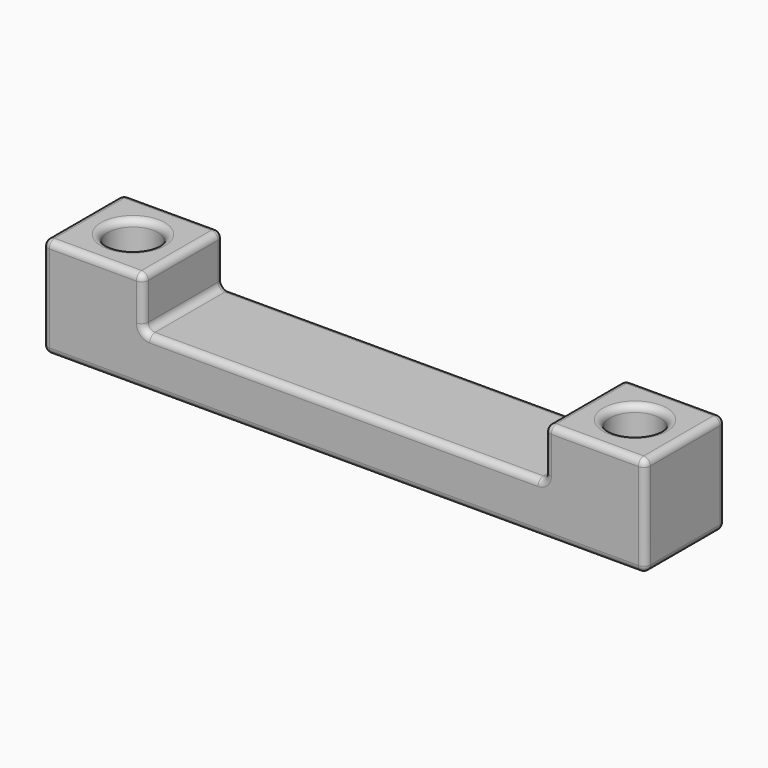
from build123d import *

# Parameters (mm, degrees)
F1_DEPTH      = 19.05
F2_R          = 4.7625
F3_DEPTH      = 19.051
F4_R          = 7.9375
F4_R_2        = 4.7625
F5_DEPTH      = 6.35
F6_T1_DEPTH   = 19.05
F6_T3_DEPTH   = 16.51
F6_T5_DEPTH   = 111.76
F6_T7_DEPTH   = 20.955
F6_T9_DEPTH   = 20.955
F6_T11_DEPTH  = 16.51
F6_T13_DEPTH  = 25.4
F6_S17_W      = 1.27
F6_S17_H      = 1.27
F6_T18_DEPTH  = 1.27
F6_S23_W      = 1.27
F6_S23_H      = 1.27
F6_T24_DEPTH  = 1.27
F6_S29_W      = 1.27
F6_S29_H      = 1.27
F6_T30_DEPTH  = 1.27
F6_S35_W      = 1.27
F6_S35_H      = 1.27
F6_T36_DEPTH  = 1.27
F6_S41_W      = 1.27
F6_S41_H      = 1.27
F6_T42_DEPTH  = 1.27
F6_S47_W      = 1.27
F6_S47_H      = 1.27
F6_T48_DEPTH  = 1.27
F6_S53_W      = 1.27
F6_S53_H      = 1.27
F6_T54_DEPTH  = 1.27
F6_S59_W      = 1.27
F6_S59_H      = 1.27
F6_T60_DEPTH  = 1.27
F6_T71_DEPTH  = 6.985
F6_T73_DEPTH  = 73.66
F6_S77_W      = 1.27
F6_S77_H      = 1.27
F6_T78_DEPTH  = 1.27
F6_S83_W      = 1.27
F6_S83_H      = 1.27
F6_T84_DEPTH  = 1.27
F6_S89_W      = 1.27
F6_S89_H      = 1.27
F6_T90_DEPTH  = 1.27
F6_S95_W      = 1.27
F6_S95_H      = 1.27
F6_T96_DEPTH  = 1.27
F6_T100_ANGLE = 90
F6_T102_ANGLE = 90
F6_T104_ANGLE = 90
F6_T106_ANGLE = 90


# Not quite as in the source:
# - a fillet or chamfer that OpenCascade refuses, or shapes differently, is made with other operations: its cross-section is extruded or revolved along the edge and cut away or added


with BuildPart() as f1:
    # F0 (on Front) → F1 (new body)
    with BuildSketch(Plane.XZ):
        Polygon((-57.15, 19.05), (-57.15, 0), (0, 0), (57.15, 0), (57.15, 19.05), (38.1, 19.05), (38.1, 9.525), (-38.1, 9.525), (-38.1, 19.05), align=None)
    extrude(amount=F1_DEPTH)

    # F2 (on face) → F3 (cut, through all)
    with BuildSketch(Plane.XY.offset(19.05)):
        with Locations((-47.625, -9.525)):
            Circle(F2_R)
        with Locations((47.625, -9.525)):
            Circle(F2_R)
    extrude(amount=-F3_DEPTH, mode=Mode.SUBTRACT)

    # F4 (on face) → F5 (cut)
    with BuildSketch(Plane(origin=(0, 0, 0), x_dir=(1, 0, 0), z_dir=(0, 0, -1))):
        with Locations((-47.625, 9.525)):
            Circle(F4_R)
        with Locations((-47.625, 9.525)):
            Circle(F4_R_2, mode=Mode.SUBTRACT)
        with Locations((47.625, 9.525)):
            Circle(F4_R)
        with Locations((47.625, 9.525)):
            Circle(F4_R_2, mode=Mode.SUBTRACT)
    extrude(amount=-F5_DEPTH, mode=Mode.SUBTRACT)

    # F6: fillet of radius 1.27 on 28 edges, made by hand

    # F6_s2 → F6_t1 (join)
    with BuildSketch(Plane.XZ):
        with BuildLine():
            ThreePointArc((38.1, 10.795), (37.7280256121, 9.8969743879), (36.83, 9.525))
            Line((36.83, 9.525), (38.1, 9.525))
            Line((38.1, 9.525), (38.1, 10.795))
        make_face()
        with BuildLine():
            ThreePointArc((-38.1, 10.795), (-37.7280256121, 9.8969743879), (-36.83, 9.525))
            Line((-36.83, 9.525), (-38.1, 9.525))
            Line((-38.1, 9.525), (-38.1, 10.795))
        make_face()
    extrude(amount=F6_T1_DEPTH)

    # F6_s4 → F6_t3 (cut)
    with BuildSketch(Plane.XY.offset(1.27)):
        with BuildLine():
            ThreePointArc((-57.15, -17.78), (-56.7780256121, -18.6780256121), (-55.88, -19.05))
            Line((-55.88, -19.05), (-57.15, -19.05))
            Line((-57.15, -19.05), (-57.15, -17.78))
        make_face()
        with BuildLine():
            ThreePointArc((55.88, -19.05), (56.7780256121, -18.6780256121), (57.15, -17.78))
            Line((57.15, -17.78), (57.15, -19.05))
            Line((57.15, -19.05), (55.88, -19.05))
        make_face()
        with BuildLine():
            ThreePointArc((-57.15, -1.27), (-56.7780256121, -0.3719743879), (-55.88, 0))
            Line((-55.88, 0), (-57.15, 0))
            Line((-57.15, 0), (-57.15, -1.27))
        make_face()
        with BuildLine():
            ThreePointArc((55.88, 0), (56.7780256121, -0.3719743879), (57.15, -1.27))
            Line((57.15, -1.27), (57.15, 0))
            Line((57.15, 0), (55.88, 0))
        make_face()
    extrude(amount=F6_T3_DEPTH, mode=Mode.SUBTRACT)

    # F6_s6 → F6_t5 (cut)
    with BuildSketch(Plane.YZ.offset(-55.88)):
        with BuildLine():
            ThreePointArc((-17.78, 0), (-18.6780256121, 0.3719743879), (-19.05, 1.27))
            Line((-19.05, 1.27), (-19.05, 0))
            Line((-19.05, 0), (-17.78, 0))
        make_face()
        with BuildLine():
            ThreePointArc((-1.27, 0), (-0.3719743879, 0.3719743879), (0, 1.27))
            Line((0, 1.27), (0, 0))
            Line((0, 0), (-1.27, 0))
        make_face()
    extrude(amount=F6_T5_DEPTH, mode=Mode.SUBTRACT)

    # F6_s8 → F6_t7 (cut)
    with BuildSketch(Plane.YZ.offset(34.925)):
        with BuildLine():
            ThreePointArc((-19.05, 17.78), (-18.6780256121, 18.6780256121), (-17.78, 19.05))
            Line((-17.78, 19.05), (-19.05, 19.05))
            Line((-19.05, 19.05), (-19.05, 17.78))
        make_face()
        with BuildLine():
            ThreePointArc((0, 17.78), (-0.3719743879, 18.6780256121), (-1.27, 19.05))
            Line((-1.27, 19.05), (0, 19.05))
            Line((0, 19.05), (0, 17.78))
        make_face()
    extrude(amount=F6_T7_DEPTH, mode=Mode.SUBTRACT)

    # F6_s10 → F6_t9 (cut)
    with BuildSketch(Plane.YZ.offset(-55.88)):
        with BuildLine():
            ThreePointArc((-17.78, 19.05), (-18.6780256121, 18.6780256121), (-19.05, 17.78))
            Line((-19.05, 17.78), (-19.05, 19.05))
            Line((-19.05, 19.05), (-17.78, 19.05))
        make_face()
        with BuildLine():
            ThreePointArc((-1.27, 19.05), (-0.3719743879, 18.6780256121), (0, 17.78))
            Line((0, 17.78), (0, 19.05))
            Line((0, 19.05), (-1.27, 19.05))
        make_face()
    extrude(amount=F6_T9_DEPTH, mode=Mode.SUBTRACT)

    # F6_s12 → F6_t11 (cut)
    with BuildSketch(Plane.XZ.offset(1.27)):
        with BuildLine():
            ThreePointArc((57.15, 17.78), (56.7780256121, 18.6780256121), (55.88, 19.05))
            Line((55.88, 19.05), (57.15, 19.05))
            Line((57.15, 19.05), (57.15, 17.78))
        make_face()
        with BuildLine():
            ThreePointArc((-57.15, 17.78), (-56.7780256121, 18.6780256121), (-55.88, 19.05))
            Line((-55.88, 19.05), (-57.15, 19.05))
            Line((-57.15, 19.05), (-57.15, 17.78))
        make_face()
        with BuildLine():
            ThreePointArc((-57.15, 1.27), (-56.7780256121, 0.3719743879), (-55.88, 0))
            Line((-55.88, 0), (-57.15, 0))
            Line((-57.15, 0), (-57.15, 1.27))
        make_face()
        with BuildLine():
            ThreePointArc((55.88, 0), (56.7780256121, 0.3719743879), (57.15, 1.27))
            Line((57.15, 1.27), (57.15, 0))
            Line((57.15, 0), (55.88, 0))
        make_face()
    extrude(amount=F6_T11_DEPTH, mode=Mode.SUBTRACT)

    # F6_s14 → F6_t13 (cut)
    with BuildSketch(Plane.XZ.offset(-3.175)):
        with BuildLine():
            ThreePointArc((39.37, 19.05), (38.4719743879, 18.6780256121), (38.1, 17.78))
            Line((38.1, 17.78), (38.1, 19.05))
            Line((38.1, 19.05), (39.37, 19.05))
        make_face()
        with BuildLine():
            ThreePointArc((-39.37, 19.05), (-38.4719743879, 18.6780256121), (-38.1, 17.78))
            Line((-38.1, 17.78), (-38.1, 19.05))
            Line((-38.1, 19.05), (-39.37, 19.05))
        make_face()
    extrude(amount=F6_T13_DEPTH, mode=Mode.SUBTRACT)


with BuildPart() as f6_tool16:
    # F6_s17 → F6_t18 (new body)
    with BuildSketch(Plane.YZ.offset(-55.88)):
        with Locations((-18.415, 18.415)):
            Rectangle(F6_S17_W, F6_S17_H)
    extrude(amount=-F6_T18_DEPTH)

    # F6_s19 → F6_t20 (revolve, cut)
    with BuildSketch(Plane(origin=(-55.88, -17.78, 17.78), x_dir=(0, 0.7071067812, -0.7071067812), z_dir=(0, 0.7071067812, 0.7071067812))):
        with BuildLine():
            ThreePointArc((0, -1.27), (1.27, 0), (0, 1.27))
            Line((0, 1.27), (0, -1.27))
        make_face()
    revolve(axis=Axis((-55.88, -17.78, 17.78), (-1, 0, 0)), mode=Mode.SUBTRACT)


with BuildPart() as f1_1:
    add(f1.part)

    # F6_t15: cut F6_tool16
    add(f6_tool16.part, mode=Mode.SUBTRACT)


with BuildPart() as f6_tool22:
    # F6_s23 → F6_t24 (new body)
    with BuildSketch(Plane.YZ.offset(-55.88)):
        with Locations((-18.415, 0.635)):
            Rectangle(F6_S23_W, F6_S23_H)
    extrude(amount=-F6_T24_DEPTH)

    # F6_s25 → F6_t26 (revolve, cut)
    with BuildSketch(Plane(origin=(-55.88, -17.78, 1.27), x_dir=(0, 0.7071067812, 0.7071067812), z_dir=(0, -0.7071067812, 0.7071067812))):
        with BuildLine():
            ThreePointArc((0, -1.27), (1.27, 0), (0, 1.27))
            Line((0, 1.27), (0, -1.27))
        make_face()
    revolve(axis=Axis((-55.88, -17.78, 1.27), (-1, 0, 0)), mode=Mode.SUBTRACT)


with BuildPart() as f1_2:
    add(f1_1.part)

    # F6_t21: cut F6_tool22
    add(f6_tool22.part, mode=Mode.SUBTRACT)


with BuildPart() as f6_tool28:
    # F6_s29 → F6_t30 (new body)
    with BuildSketch(Plane.XY.offset(1.27)):
        with Locations((56.515, -18.415)):
            Rectangle(F6_S29_W, F6_S29_H)
    extrude(amount=-F6_T30_DEPTH)

    # F6_s31 → F6_t32 (revolve, cut)
    with BuildSketch(Plane(origin=(55.88, -17.78, 1.27), x_dir=(-0.7071067812, 0.7071067812, 0), z_dir=(-0.7071067812, -0.7071067812, 0))):
        with BuildLine():
            ThreePointArc((0, -1.27), (1.27, 0), (0, 1.27))
            Line((0, 1.27), (0, -1.27))
        make_face()
    revolve(axis=Axis((55.88, -17.78, 1.27), (0, 0, -1)), mode=Mode.SUBTRACT)


with BuildPart() as f1_3:
    add(f1_2.part)

    # F6_t27: cut F6_tool28
    add(f6_tool28.part, mode=Mode.SUBTRACT)


with BuildPart() as f6_tool34:
    # F6_s35 → F6_t36 (new body)
    with BuildSketch(Plane.XY.offset(17.78)):
        with Locations((56.515, -18.415)):
            Rectangle(F6_S35_W, F6_S35_H)
    extrude(amount=F6_T36_DEPTH)

    # F6_s37 → F6_t38 (revolve, cut)
    with BuildSketch(Plane(origin=(55.88, -17.78, 17.78), x_dir=(-0.7071067812, 0.7071067812, 0), z_dir=(0.7071067812, 0.7071067812, 0))):
        with BuildLine():
            ThreePointArc((0, -1.27), (1.27, 0), (0, 1.27))
            Line((0, 1.27), (0, -1.27))
        make_face()
    revolve(axis=Axis((55.88, -17.78, 17.78), (0, 0, 1)), mode=Mode.SUBTRACT)


with BuildPart() as f1_4:
    add(f1_3.part)

    # F6_t33: cut F6_tool34
    add(f6_tool34.part, mode=Mode.SUBTRACT)


with BuildPart() as f6_tool40:
    # F6_s41 → F6_t42 (new body)
    with BuildSketch(Plane.YZ.offset(-55.88)):
        with Locations((-0.635, 18.415)):
            Rectangle(F6_S41_W, F6_S41_H)
    extrude(amount=-F6_T42_DEPTH)

    # F6_s43 → F6_t44 (revolve, cut)
    with BuildSketch(Plane(origin=(-55.88, -1.27, 17.78), x_dir=(0, -0.7071067812, -0.7071067812), z_dir=(0, 0.7071067812, -0.7071067812))):
        with BuildLine():
            ThreePointArc((0, -1.27), (1.27, 0), (0, 1.27))
            Line((0, 1.27), (0, -1.27))
        make_face()
    revolve(axis=Axis((-55.88, -1.27, 17.78), (-1, 0, 0)), mode=Mode.SUBTRACT)


with BuildPart() as f1_5:
    add(f1_4.part)

    # F6_t39: cut F6_tool40
    add(f6_tool40.part, mode=Mode.SUBTRACT)


with BuildPart() as f6_tool46:
    # F6_s47 → F6_t48 (new body)
    with BuildSketch(Plane.YZ.offset(-55.88)):
        with Locations((-0.635, 0.635)):
            Rectangle(F6_S47_W, F6_S47_H)
    extrude(amount=-F6_T48_DEPTH)

    # F6_s49 → F6_t50 (revolve, cut)
    with BuildSketch(Plane(origin=(-55.88, -1.27, 1.27), x_dir=(0, -0.7071067812, 0.7071067812), z_dir=(0, -0.7071067812, -0.7071067812))):
        with BuildLine():
            ThreePointArc((0, -1.27), (1.27, 0), (0, 1.27))
            Line((0, 1.27), (0, -1.27))
        make_face()
    revolve(axis=Axis((-55.88, -1.27, 1.27), (-1, 0, 0)), mode=Mode.SUBTRACT)


with BuildPart() as f1_6:
    add(f1_5.part)

    # F6_t45: cut F6_tool46
    add(f6_tool46.part, mode=Mode.SUBTRACT)


with BuildPart() as f6_tool52:
    # F6_s53 → F6_t54 (new body)
    with BuildSketch(Plane.XY.offset(1.27)):
        with Locations((56.515, -0.635)):
            Rectangle(F6_S53_W, F6_S53_H)
    extrude(amount=-F6_T54_DEPTH)

    # F6_s55 → F6_t56 (revolve, cut)
    with BuildSketch(Plane(origin=(55.88, -1.27, 1.27), x_dir=(-0.7071067812, -0.7071067812, 0), z_dir=(0.7071067812, -0.7071067812, 0))):
        with BuildLine():
            ThreePointArc((0, -1.27), (1.27, 0), (0, 1.27))
            Line((0, 1.27), (0, -1.27))
        make_face()
    revolve(axis=Axis((55.88, -1.27, 1.27), (0, 0, -1)), mode=Mode.SUBTRACT)


with BuildPart() as f1_7:
    add(f1_6.part)

    # F6_t51: cut F6_tool52
    add(f6_tool52.part, mode=Mode.SUBTRACT)


with BuildPart() as f6_tool58:
    # F6_s59 → F6_t60 (new body)
    with BuildSketch(Plane.XY.offset(17.78)):
        with Locations((56.515, -0.635)):
            Rectangle(F6_S59_W, F6_S59_H)
    extrude(amount=F6_T60_DEPTH)

    # F6_s61 → F6_t62 (revolve, cut)
    with BuildSketch(Plane(origin=(55.88, -1.27, 17.78), x_dir=(-0.7071067812, -0.7071067812, 0), z_dir=(-0.7071067812, 0.7071067812, 0))):
        with BuildLine():
            ThreePointArc((0, -1.27), (1.27, 0), (0, 1.27))
            Line((0, 1.27), (0, -1.27))
        make_face()
    revolve(axis=Axis((55.88, -1.27, 17.78), (0, 0, 1)), mode=Mode.SUBTRACT)


with BuildPart() as f1_8:
    add(f1_7.part)

    # F6_t57: cut F6_tool58
    add(f6_tool58.part, mode=Mode.SUBTRACT)

    # F6_s63 → F6_t64 (revolve, cut)
    with BuildSketch(Plane.XZ.offset(9.525)):
        with BuildLine():
            ThreePointArc((53.6575, 19.05), (52.7594743879, 18.6780256121), (52.3875, 17.78))
            Line((52.3875, 17.78), (52.3875, 19.05))
            Line((52.3875, 19.05), (53.6575, 19.05))
        make_face()
    revolve(axis=Axis((47.625, -9.525, 19.05), (0, 0, 1)), mode=Mode.SUBTRACT)

    # F6_s65 → F6_t66 (revolve, cut)
    with BuildSketch(Plane.XZ.offset(9.525)):
        with BuildLine():
            ThreePointArc((-41.5925, 19.05), (-42.4905256121, 18.6780256121), (-42.8625, 17.78))
            Line((-42.8625, 17.78), (-42.8625, 19.05))
            Line((-42.8625, 19.05), (-41.5925, 19.05))
        make_face()
    revolve(axis=Axis((-47.625, -9.525, 19.05), (0, 0, 1)), mode=Mode.SUBTRACT)

    # F6_s67 → F6_t68 (revolve, cut)
    with BuildSketch(Plane.XZ.offset(9.525)):
        with BuildLine():
            ThreePointArc((-38.4175, 0), (-39.3155256121, 0.3719743879), (-39.6875, 1.27))
            Line((-39.6875, 1.27), (-39.6875, 0))
            Line((-39.6875, 0), (-38.4175, 0))
        make_face()
    revolve(axis=Axis((-47.625, -9.525, 0), (0, 0, -1)), mode=Mode.SUBTRACT)

    # F6_s69 → F6_t70 (revolve, cut)
    with BuildSketch(Plane.XZ.offset(9.525)):
        with BuildLine():
            ThreePointArc((56.8325, 0), (55.9344743879, 0.3719743879), (55.5625, 1.27))
            Line((55.5625, 1.27), (55.5625, 0))
            Line((55.5625, 0), (56.8325, 0))
        make_face()
    revolve(axis=Axis((47.625, -9.525, 0), (0, 0, -1)), mode=Mode.SUBTRACT)

    # F6_s72 → F6_t71 (cut)
    with BuildSketch(Plane.XY.offset(10.795)):
        with BuildLine():
            ThreePointArc((39.37, -19.05), (38.4719743879, -18.6780256121), (38.1, -17.78))
            Line((38.1, -17.78), (38.1, -19.05))
            Line((38.1, -19.05), (39.37, -19.05))
        make_face()
        with BuildLine():
            ThreePointArc((-39.37, -19.05), (-38.4719743879, -18.6780256121), (-38.1, -17.78))
            Line((-38.1, -17.78), (-38.1, -19.05))
            Line((-38.1, -19.05), (-39.37, -19.05))
        make_face()
        with BuildLine():
            ThreePointArc((39.37, 0), (38.4719743879, -0.3719743879), (38.1, -1.27))
            Line((38.1, -1.27), (38.1, 0))
            Line((38.1, 0), (39.37, 0))
        make_face()
        with BuildLine():
            ThreePointArc((-39.37, 0), (-38.4719743879, -0.3719743879), (-38.1, -1.27))
            Line((-38.1, -1.27), (-38.1, 0))
            Line((-38.1, 0), (-39.37, 0))
        make_face()
    extrude(amount=F6_T71_DEPTH, mode=Mode.SUBTRACT)

    # F6_s74 → F6_t73 (cut)
    with BuildSketch(Plane.YZ.offset(-36.83)):
        with BuildLine():
            ThreePointArc((-19.05, 8.255), (-18.6780256121, 9.1530256121), (-17.78, 9.525))
            Line((-17.78, 9.525), (-19.05, 9.525))
            Line((-19.05, 9.525), (-19.05, 8.255))
        make_face()
        with BuildLine():
            ThreePointArc((0, 8.255), (-0.3719743879, 9.1530256121), (-1.27, 9.525))
            Line((-1.27, 9.525), (0, 9.525))
            Line((0, 9.525), (0, 8.255))
        make_face()
    extrude(amount=F6_T73_DEPTH, mode=Mode.SUBTRACT)


with BuildPart() as f6_tool76:
    # F6_s77 → F6_t78 (new body)
    with BuildSketch(Plane.XZ.offset(1.27)):
        with Locations((-38.735, 18.415)):
            Rectangle(F6_S77_W, F6_S77_H)
    extrude(amount=-F6_T78_DEPTH)

    # F6_s79 → F6_t80 (revolve, cut)
    with BuildSketch(Plane(origin=(-39.37, -1.27, 17.78), x_dir=(-0.7071067812, 0, -0.7071067812), z_dir=(0.7071067812, 0, -0.7071067812))):
        with BuildLine():
            ThreePointArc((0, -1.27), (1.27, 0), (0, 1.27))
            Line((0, 1.27), (0, -1.27))
        make_face()
    revolve(axis=Axis((-39.37, -1.27, 17.78), (0, 1, 0)), mode=Mode.SUBTRACT)


with BuildPart() as f1_9:
    add(f1_8.part)

    # F6_t75: cut F6_tool76
    add(f6_tool76.part, mode=Mode.SUBTRACT)


with BuildPart() as f6_tool82:
    # F6_s83 → F6_t84 (new body)
    with BuildSketch(Plane.XZ.offset(1.27)):
        with Locations((38.735, 18.415)):
            Rectangle(F6_S83_W, F6_S83_H)
    extrude(amount=-F6_T84_DEPTH)

    # F6_s85 → F6_t86 (revolve, cut)
    with BuildSketch(Plane(origin=(39.37, -1.27, 17.78), x_dir=(0.7071067812, 0, -0.7071067812), z_dir=(0.7071067812, 0, 0.7071067812))):
        with BuildLine():
            ThreePointArc((0, -1.27), (1.27, 0), (0, 1.27))
            Line((0, 1.27), (0, -1.27))
        make_face()
    revolve(axis=Axis((39.37, -1.27, 17.78), (0, 1, 0)), mode=Mode.SUBTRACT)


with BuildPart() as f1_10:
    add(f1_9.part)

    # F6_t81: cut F6_tool82
    add(f6_tool82.part, mode=Mode.SUBTRACT)


with BuildPart() as f6_tool88:
    # F6_s89 → F6_t90 (new body)
    with BuildSketch(Plane.XZ.offset(17.78)):
        with Locations((-38.735, 18.415)):
            Rectangle(F6_S89_W, F6_S89_H)
    extrude(amount=F6_T90_DEPTH)

    # F6_s91 → F6_t92 (revolve, cut)
    with BuildSketch(Plane(origin=(-39.37, -17.78, 17.78), x_dir=(-0.7071067812, 0, -0.7071067812), z_dir=(-0.7071067812, 0, 0.7071067812))):
        with BuildLine():
            ThreePointArc((0, -1.27), (1.27, 0), (0, 1.27))
            Line((0, 1.27), (0, -1.27))
        make_face()
    revolve(axis=Axis((-39.37, -17.78, 17.78), (0, -1, 0)), mode=Mode.SUBTRACT)


with BuildPart() as f1_11:
    add(f1_10.part)

    # F6_t87: cut F6_tool88
    add(f6_tool88.part, mode=Mode.SUBTRACT)


with BuildPart() as f6_tool94:
    # F6_s95 → F6_t96 (new body)
    with BuildSketch(Plane.XZ.offset(17.78)):
        with Locations((38.735, 18.415)):
            Rectangle(F6_S95_W, F6_S95_H)
    extrude(amount=F6_T96_DEPTH)

    # F6_s97 → F6_t98 (revolve, cut)
    with BuildSketch(Plane(origin=(39.37, -17.78, 17.78), x_dir=(0.7071067812, 0, -0.7071067812), z_dir=(-0.7071067812, 0, -0.7071067812))):
        with BuildLine():
            ThreePointArc((0, -1.27), (1.27, 0), (0, 1.27))
            Line((0, 1.27), (0, -1.27))
        make_face()
    revolve(axis=Axis((39.37, -17.78, 17.78), (0, -1, 0)), mode=Mode.SUBTRACT)


with BuildPart() as f1_12:
    add(f1_11.part)

    # F6_t93: cut F6_tool94
    add(f6_tool94.part, mode=Mode.SUBTRACT)

    # F6_s99 → F6_t100 (revolve, cut)
    with BuildSketch(Plane.XY.offset(10.795)):
        with BuildLine():
            ThreePointArc((-39.37, 0), (-38.4719743879, -0.3719743879), (-38.1, -1.27))
            Line((-38.1, -1.27), (-38.1, 0))
            Line((-38.1, 0), (-39.37, 0))
        make_face()
    revolve(axis=Axis((-36.83, 0, 10.795), (0, -1, 0)), revolution_arc=F6_T100_ANGLE, mode=Mode.SUBTRACT)

    # F6_s101 → F6_t102 (revolve, cut)
    with BuildSketch(Plane.XY.offset(10.795)):
        with BuildLine():
            ThreePointArc((39.37, 0), (38.4719743879, -0.3719743879), (38.1, -1.27))
            Line((38.1, -1.27), (38.1, 0))
            Line((38.1, 0), (39.37, 0))
        make_face()
    revolve(axis=Axis((36.83, 0, 10.795), (0, 1, 0)), revolution_arc=F6_T102_ANGLE, mode=Mode.SUBTRACT)

    # F6_s103 → F6_t104 (revolve, cut)
    with BuildSketch(Plane.XY.offset(10.795)):
        with BuildLine():
            ThreePointArc((-39.37, -19.05), (-38.4719743879, -18.6780256121), (-38.1, -17.78))
            Line((-38.1, -17.78), (-38.1, -19.05))
            Line((-38.1, -19.05), (-39.37, -19.05))
        make_face()
    revolve(axis=Axis((-36.83, -19.05, 10.795), (0, -1, 0)), revolution_arc=F6_T104_ANGLE, mode=Mode.SUBTRACT)

    # F6_s105 → F6_t106 (revolve, cut)
    with BuildSketch(Plane.XY.offset(10.795)):
        with BuildLine():
            ThreePointArc((39.37, -19.05), (38.4719743879, -18.6780256121), (38.1, -17.78))
            Line((38.1, -17.78), (38.1, -19.05))
            Line((38.1, -19.05), (39.37, -19.05))
        make_face()
    revolve(axis=Axis((36.83, -19.05, 10.795), (0, 1, 0)), revolution_arc=F6_T106_ANGLE, mode=Mode.SUBTRACT)


solid = f1_12.part
